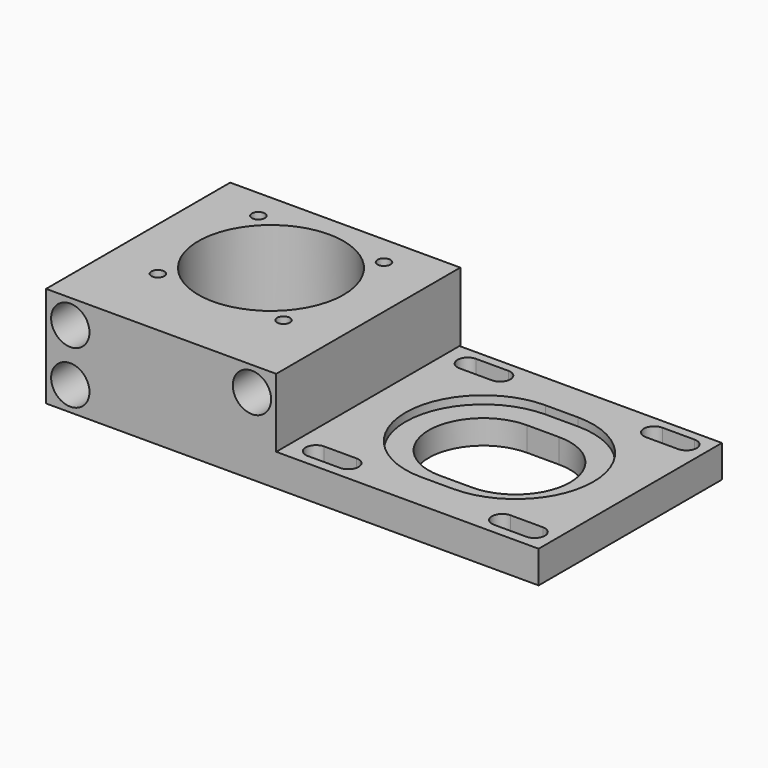
from build123d import *

# Parameters (mm, degrees)
F0_W     = 57
F0_H     = 57
F0_R     = 1.6
F0_R_2   = 18
F0_W_2   = 65
F1_DEPTH = 25
F2_DEPTH = 17
F3_DEPTH = 19
F4_R     = 2.55
F5_DEPTH = 60
F4_R_2   = 4.75
F6_DEPTH = 20
F7_DEPTH = 15
F8_W     = 65
F8_H     = 8
F9_DEPTH = 0.25
F10_SIZE = 0.2


# Not quite as in the source:
# - a feature names something its author has since deleted; it is built from what else it names


with BuildPart() as f1:
    # F0 (on Top) → F1 (new body)
    with BuildSketch(Plane.XY):
        with Locations((28.5, -28.5)):
            Rectangle(F0_W, F0_H)
        with Locations((12.9436508139, -38.5563491861)):
            Circle(F0_R, mode=Mode.SUBTRACT)
        with Locations((44.0563491861, -38.5563491861)):
            Circle(F0_R, mode=Mode.SUBTRACT)
        with Locations((28.5, -23)):
            Circle(F0_R_2, mode=Mode.SUBTRACT)
        with Locations((12.9436508139, -7.4436508139)):
            Circle(F0_R, mode=Mode.SUBTRACT)
        with Locations((44.0563491861, -7.4436508139)):
            Circle(F0_R, mode=Mode.SUBTRACT)
        with Locations((89.5, -28.5)):
            Rectangle(F0_W_2, F0_H)
        with BuildLine():
            Line((62.86, -49.45), (70.86, -49.45))
            ThreePointArc((70.86, -49.45), (73.41, -52), (70.86, -54.55))
            Line((70.86, -54.55), (62.86, -54.55))
            ThreePointArc((62.86, -54.55), (60.31, -52), (62.86, -49.45))
        make_face(mode=Mode.SUBTRACT)
        with BuildLine():
            Line((117, -54.55), (109, -54.55))
            ThreePointArc((109, -54.55), (106.45, -52), (109, -49.45))
            Line((109, -49.45), (117, -49.45))
            ThreePointArc((117, -49.45), (119.55, -52), (117, -54.55))
        make_face(mode=Mode.SUBTRACT)
        with BuildLine():
            Line((85.5, -9.25), (93.5, -9.25))
            ThreePointArc((93.5, -9.25), (112.75, -28.5), (93.5, -47.75))
            Line((93.5, -47.75), (85.5, -47.75))
            ThreePointArc((85.5, -47.75), (66.25, -28.5), (85.5, -9.25))
        make_face(mode=Mode.SUBTRACT)
        with BuildLine():
            Line((62.86, -2.45), (70.86, -2.45))
            ThreePointArc((70.86, -2.45), (73.41, -5), (70.86, -7.55))
            Line((70.86, -7.55), (62.86, -7.55))
            ThreePointArc((62.86, -7.55), (60.31, -5), (62.86, -2.45))
        make_face(mode=Mode.SUBTRACT)
        with BuildLine():
            Line((117, -7.55), (109, -7.55))
            ThreePointArc((109, -7.55), (106.45, -5), (109, -2.45))
            Line((109, -2.45), (117, -2.45))
            ThreePointArc((117, -2.45), (119.55, -5), (117, -7.55))
        make_face(mode=Mode.SUBTRACT)
        with Locations((12.9436508139, -7.4436508139)):
            Circle(F0_R)
        with Locations((44.0563491861, -7.4436508139)):
            Circle(F0_R)
        with Locations((44.0563491861, -38.5563491861)):
            Circle(F0_R)
        with Locations((12.9436508139, -38.5563491861)):
            Circle(F0_R)
        with BuildLine():
            ThreePointArc((93.5, -47.75), (112.75, -28.5), (93.5, -9.25))
            Line((93.5, -9.25), (85.5, -9.25))
            ThreePointArc((85.5, -9.25), (66.25, -28.5), (85.5, -47.75))
            Line((85.5, -47.75), (93.5, -47.75))
        make_face()
        with BuildLine():
            Line((85.5, -15), (93.5, -15))
            ThreePointArc((93.5, -15), (107, -28.5), (93.5, -42))
            Line((93.5, -42), (85.5, -42))
            ThreePointArc((85.5, -42), (72, -28.5), (85.5, -15))
        make_face(mode=Mode.SUBTRACT)
    extrude(amount=-F1_DEPTH)

    # F0 (on Top) → F2 (cut)
    with BuildSketch(Plane.XY):
        with Locations((89.5, -28.5)):
            Rectangle(F0_W_2, F0_H)
        with BuildLine():
            Line((62.86, -49.45), (70.86, -49.45))
            ThreePointArc((70.86, -49.45), (73.41, -52), (70.86, -54.55))
            Line((70.86, -54.55), (62.86, -54.55))
            ThreePointArc((62.86, -54.55), (60.31, -52), (62.86, -49.45))
        make_face(mode=Mode.SUBTRACT)
        with BuildLine():
            Line((117, -54.55), (109, -54.55))
            ThreePointArc((109, -54.55), (106.45, -52), (109, -49.45))
            Line((109, -49.45), (117, -49.45))
            ThreePointArc((117, -49.45), (119.55, -52), (117, -54.55))
        make_face(mode=Mode.SUBTRACT)
        with BuildLine():
            Line((85.5, -9.25), (93.5, -9.25))
            ThreePointArc((93.5, -9.25), (112.75, -28.5), (93.5, -47.75))
            Line((93.5, -47.75), (85.5, -47.75))
            ThreePointArc((85.5, -47.75), (66.25, -28.5), (85.5, -9.25))
        make_face(mode=Mode.SUBTRACT)
        with BuildLine():
            Line((62.86, -2.45), (70.86, -2.45))
            ThreePointArc((70.86, -2.45), (73.41, -5), (70.86, -7.55))
            Line((70.86, -7.55), (62.86, -7.55))
            ThreePointArc((62.86, -7.55), (60.31, -5), (62.86, -2.45))
        make_face(mode=Mode.SUBTRACT)
        with BuildLine():
            Line((117, -7.55), (109, -7.55))
            ThreePointArc((109, -7.55), (106.45, -5), (109, -2.45))
            Line((109, -2.45), (117, -2.45))
            ThreePointArc((117, -2.45), (119.55, -5), (117, -7.55))
        make_face(mode=Mode.SUBTRACT)
    extrude(amount=-F2_DEPTH, mode=Mode.SUBTRACT)

    # F0 (on Top) → F3 (cut)
    with BuildSketch(Plane.XY):
        with BuildLine():
            ThreePointArc((93.5, -47.75), (112.75, -28.5), (93.5, -9.25))
            Line((93.5, -9.25), (85.5, -9.25))
            ThreePointArc((85.5, -9.25), (66.25, -28.5), (85.5, -47.75))
            Line((85.5, -47.75), (93.5, -47.75))
        make_face()
        with BuildLine():
            Line((85.5, -15), (93.5, -15))
            ThreePointArc((93.5, -15), (107, -28.5), (93.5, -42))
            Line((93.5, -42), (85.5, -42))
            ThreePointArc((85.5, -42), (72, -28.5), (85.5, -15))
        make_face(mode=Mode.SUBTRACT)
        with BuildLine():
            ThreePointArc((93.5, -42), (107, -28.5), (93.5, -15))
            Line((93.5, -15), (85.5, -15))
            ThreePointArc((85.5, -15), (72, -28.5), (85.5, -42))
            Line((85.5, -42), (93.5, -42))
        make_face()
    extrude(amount=-F3_DEPTH, mode=Mode.SUBTRACT)

    # F4 (on face) → F5 (cut)
    with BuildSketch(Plane.XZ.offset(57)):
        with Locations((6, -6)):
            Circle(F4_R)
        with Locations((6, -19)):
            Circle(F4_R)
        with Locations((51, -6)):
            Circle(F4_R)
    extrude(amount=-F5_DEPTH, mode=Mode.SUBTRACT)

    # F4 (on face) → F6 (cut)
    with BuildSketch(Plane.XZ.offset(57)):
        with Locations((6, -6)):
            Circle(F4_R_2)
        with Locations((6, -6)):
            Circle(F4_R, mode=Mode.SUBTRACT)
        with Locations((6, -19)):
            Circle(F4_R_2)
        with Locations((6, -19)):
            Circle(F4_R, mode=Mode.SUBTRACT)
        with Locations((51, -6)):
            Circle(F4_R_2)
        with Locations((51, -6)):
            Circle(F4_R, mode=Mode.SUBTRACT)
    extrude(amount=-F6_DEPTH, mode=Mode.SUBTRACT)

    # F0 (on Top) → F7 (cut)
    with BuildSketch(Plane.XY):
        with Locations((44.0563491861, -7.4436508139)):
            Circle(F0_R)
        with Locations((44.0563491861, -38.5563491861)):
            Circle(F0_R)
        with Locations((12.9436508139, -38.5563491861)):
            Circle(F0_R)
        with Locations((12.9436508139, -7.4436508139)):
            Circle(F0_R)
    extrude(amount=-F7_DEPTH, mode=Mode.SUBTRACT)

    # F8 (on face) → F9 (cut)
    with BuildSketch(Plane(origin=(0, 0, 0), x_dir=(-1, 0, 0), z_dir=(0, 1, 0))):
        with Locations((-89.5, -21)):
            Rectangle(F8_W, F8_H)
    extrude(amount=-F9_DEPTH, mode=Mode.SUBTRACT)

    # F10
    f10_edges = [f1.edges().sort_by_distance(p)[0] for p in [
        (48.45, 0, -6),
        (3.45, 0, -6),
        (3.45, 0, -19),
    ]]
    chamfer(f10_edges, length=F10_SIZE)


solid = f1.part
